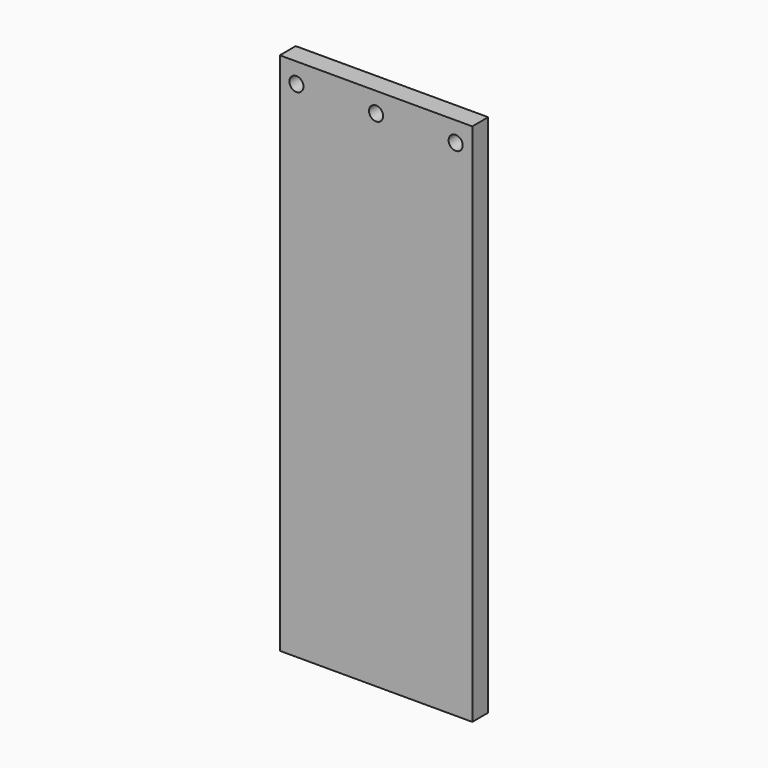
from build123d import *

# Parameters (mm, degrees)
F0_W     = 92.075
F0_H     = 250.825
F1_DEPTH = 9.525
F3_D     = 6.7564
F5_D     = 5
F5_DEPTH = 28.4
F5_TIP   = 1.5021515476


# Not quite as in the source:
# - a feature names something its author has since deleted; it is built from what else it names


with BuildPart() as f1:
    # F0 (on Front) → F1 (new body)
    with BuildSketch(Plane.XZ):
        with Locations((46.0375, 125.4125)):
            Rectangle(F0_W, F0_H)
    extrude(amount=-F1_DEPTH)

    # F3 (through all)
    with Locations(Plane.XZ):
        with Locations((46.0375, 241.3), (84.1375, 241.3), (7.9375, 241.3)):
            Hole(F3_D / 2)

    # F5
    with Locations(Plane(origin=(0, 0, 0), x_dir=(1, 0, 0), z_dir=(0, 0, -1))):
        with Locations((7.9375, -4.7625), (33.3375, -4.7625), (58.7375, -4.7625), (84.1375, -4.7625), (109.5375, -4.7625), (134.9375, -4.7625)):
            Hole(F5_D / 2, depth=F5_DEPTH)
            with Locations((0, 0, -(F5_DEPTH + F5_TIP / 2))):  # 118° drill point
                Cone(0, F5_D / 2, F5_TIP, mode=Mode.SUBTRACT)


solid = f1.part
